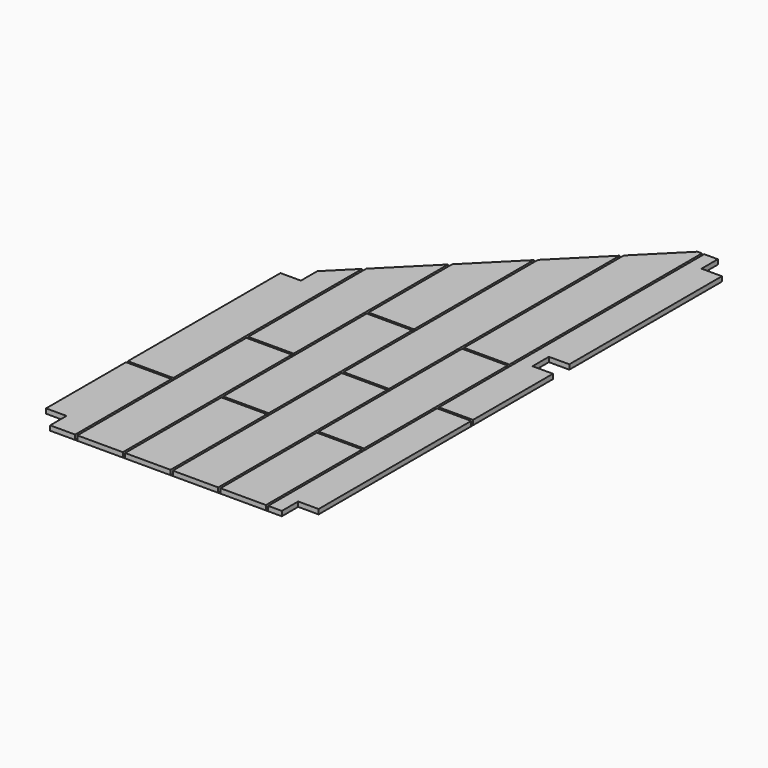
from build123d import *

# Parameters (mm, degrees)
F0_W     = 20
F0_H     = 93
F0_H_2   = 79
F0_H_3   = 53
F0_H_4   = 1
F0_W_2   = 15
F0_W_3   = 2
F0_H_5   = 9
F0_W_4   = 1
F0_W_5   = 6
F1_DEPTH = 0.1
F2_DEPTH = 2


# Not quite as in the source:
# - a feature names something its author has since deleted; it is built from what else it names


with BuildPart() as f1:
    # F0 (on Top) → F1 (new body)
    with BuildSketch(Plane.XY):
        Polygon((-134.4656153619, 144.6975417137), (-143.4656153619, 144.6975417137), (-143.4656153619, 104.6975417137), (-143.4656153619, 95.6975417137), (-143.4656153619, 64.6975417137), (-143.4656153619, 60.6975417137), (-123.4656153619, 60.6975417137), (-123.4656153619, 164.6975417137), (-134.4656153619, 153.6975417137), align=None)
        Polygon((-123.4656153619, 6.6975417137), (-123.4656153619, 59.6975417137), (-143.4656153619, 59.6975417137), (-143.4656153619, 55.6975417137), (-143.4656153619, 15.6975417137), (-134.4656153619, 15.6975417137), (-134.4656153619, 6.6975417137), align=None)
        with Locations((-112.4656153619, 53.1975417137)):
            Rectangle(F0_W, F0_H)
        Polygon((-102.4656153619, 185.6975417137), (-122.4656153619, 165.6975417137), (-122.4656153619, 100.6975417137), (-102.4656153619, 100.6975417137), align=None)
        Polygon((-81.4656153619, 140.6975417137), (-81.4656153619, 206.6975417137), (-101.4656153619, 186.6975417137), (-101.4656153619, 140.6975417137), align=None)
        with Locations((-91.4656153619, 100.1975417137)):
            Rectangle(F0_W, F0_H_2)
        with Locations((-91.4656153619, 33.1975417137)):
            Rectangle(F0_W, F0_H_3)
        Polygon((-60.4656153619, 100.6975417137), (-60.4656153619, 227.6975417137), (-80.4656153619, 207.6975417137), (-80.4656153619, 100.6975417137), align=None)
        with Locations((-70.4656153619, 53.1975417137)):
            Rectangle(F0_W, F0_H)
        Polygon((-41.4656153619, 237.6975417137), (-41.4656153619, 246.6975417137), (-59.4656153619, 228.6975417137), (-59.4656153619, 140.6975417137), (-39.4656153619, 140.6975417137), (-39.4656153619, 237.6975417137), align=None)
        with Locations((-49.4656153619, 100.1975417137)):
            Rectangle(F0_W, F0_H_2)
        with Locations((-49.4656153619, 33.1975417137)):
            Rectangle(F0_W, F0_H_3)
        with Locations((-133.4656153619, 60.1975417137)):
            Rectangle(F0_W, F0_H_4)
        Polygon((-122.4656153619, 165.6975417137), (-123.4656153619, 164.6975417137), (-123.4656153619, 60.6975417137), (-123.4656153619, 59.6975417137), (-123.4656153619, 6.6975417137), (-122.4656153619, 6.6975417137), (-122.4656153619, 99.6975417137), (-122.4656153619, 100.6975417137), align=None)
        with Locations((-112.4656153619, 100.1975417137)):
            Rectangle(F0_W, F0_H_4)
        Polygon((-101.4656153619, 186.6975417137), (-102.4656153619, 185.6975417137), (-102.4656153619, 100.6975417137), (-102.4656153619, 99.6975417137), (-102.4656153619, 6.6975417137), (-101.4656153619, 6.6975417137), (-101.4656153619, 59.6975417137), (-101.4656153619, 60.6975417137), (-101.4656153619, 139.6975417137), (-101.4656153619, 140.6975417137), align=None)
        with Locations((-91.4656153619, 140.1975417137)):
            Rectangle(F0_W, F0_H_4)
        Polygon((-80.4656153619, 100.6975417137), (-80.4656153619, 207.6975417137), (-81.4656153619, 206.6975417137), (-81.4656153619, 140.6975417137), (-81.4656153619, 139.6975417137), (-81.4656153619, 60.6975417137), (-81.4656153619, 59.6975417137), (-81.4656153619, 6.6975417137), (-80.4656153619, 6.6975417137), (-80.4656153619, 99.6975417137), align=None)
        with Locations((-70.4656153619, 100.1975417137)):
            Rectangle(F0_W, F0_H_4)
        Polygon((-59.4656153619, 140.6975417137), (-59.4656153619, 228.6975417137), (-60.4656153619, 227.6975417137), (-60.4656153619, 100.6975417137), (-60.4656153619, 99.6975417137), (-60.4656153619, 6.6975417137), (-59.4656153619, 6.6975417137), (-59.4656153619, 59.6975417137), (-59.4656153619, 60.6975417137), (-59.4656153619, 139.6975417137), align=None)
        with Locations((-49.4656153619, 60.1975417137)):
            Rectangle(F0_W, F0_H_4)
        with Locations((-49.4656153619, 140.1975417137)):
            Rectangle(F0_W, F0_H_4)
        with Locations((-91.4656153619, 60.1975417137)):
            Rectangle(F0_W, F0_H_4)
        Polygon((-38.4656153619, 237.6975417137), (-39.4656153619, 237.6975417137), (-39.4656153619, 140.6975417137), (-39.4656153619, 139.6975417137), (-39.4656153619, 60.6975417137), (-39.4656153619, 59.6975417137), (-39.4656153619, 6.6975417137), (-38.4656153619, 6.6975417137), (-38.4656153619, 99.6975417137), (-38.4656153619, 100.6975417137), align=None)
        Polygon((-23.4656153619, 99.6975417137), (-38.4656153619, 99.6975417137), (-38.4656153619, 6.6975417137), (-32.4656153619, 6.6975417137), (-32.4656153619, 15.6975417137), (-23.4656153619, 15.6975417137), align=None)
        Polygon((-32.4656153619, 237.6975417137), (-38.4656153619, 237.6975417137), (-38.4656153619, 100.6975417137), (-23.4656153619, 100.6975417137), (-23.4656153619, 144.6975417137), (-32.4656153619, 144.6975417137), (-32.4656153619, 153.6975417137), (-23.4656153619, 153.6975417137), (-23.4656153619, 237.6975417137), align=None)
        with Locations((-30.9656153619, 100.1975417137)):
            Rectangle(F0_W_2, F0_H_4)
        with Locations((-40.4656153619, 242.1975417137)):
            Rectangle(F0_W_3, F0_H_5)
        with Locations((-38.9656153619, 242.1975417137)):
            Rectangle(F0_W_4, F0_H_5)
        with Locations((-35.4656153619, 242.1975417137)):
            Rectangle(F0_W_5, F0_H_5)
    extrude(amount=-F1_DEPTH)

    # F0 (on Top) → F2 (join)
    with BuildSketch(Plane.XY):
        Polygon((-134.4656153619, 144.6975417137), (-143.4656153619, 144.6975417137), (-143.4656153619, 104.6975417137), (-143.4656153619, 95.6975417137), (-143.4656153619, 64.6975417137), (-143.4656153619, 60.6975417137), (-123.4656153619, 60.6975417137), (-123.4656153619, 164.6975417137), (-134.4656153619, 153.6975417137), align=None)
        Polygon((-123.4656153619, 6.6975417137), (-123.4656153619, 59.6975417137), (-143.4656153619, 59.6975417137), (-143.4656153619, 55.6975417137), (-143.4656153619, 15.6975417137), (-134.4656153619, 15.6975417137), (-134.4656153619, 6.6975417137), align=None)
        with Locations((-112.4656153619, 53.1975417137)):
            Rectangle(F0_W, F0_H)
        Polygon((-102.4656153619, 185.6975417137), (-122.4656153619, 165.6975417137), (-122.4656153619, 100.6975417137), (-102.4656153619, 100.6975417137), align=None)
        Polygon((-81.4656153619, 140.6975417137), (-81.4656153619, 206.6975417137), (-101.4656153619, 186.6975417137), (-101.4656153619, 140.6975417137), align=None)
        with Locations((-91.4656153619, 100.1975417137)):
            Rectangle(F0_W, F0_H_2)
        with Locations((-91.4656153619, 33.1975417137)):
            Rectangle(F0_W, F0_H_3)
        with Locations((-70.4656153619, 53.1975417137)):
            Rectangle(F0_W, F0_H)
        Polygon((-60.4656153619, 100.6975417137), (-60.4656153619, 227.6975417137), (-80.4656153619, 207.6975417137), (-80.4656153619, 100.6975417137), align=None)
        Polygon((-41.4656153619, 237.6975417137), (-41.4656153619, 246.6975417137), (-59.4656153619, 228.6975417137), (-59.4656153619, 140.6975417137), (-39.4656153619, 140.6975417137), (-39.4656153619, 237.6975417137), align=None)
        with Locations((-49.4656153619, 100.1975417137)):
            Rectangle(F0_W, F0_H_2)
        with Locations((-49.4656153619, 33.1975417137)):
            Rectangle(F0_W, F0_H_3)
        Polygon((-23.4656153619, 99.6975417137), (-38.4656153619, 99.6975417137), (-38.4656153619, 6.6975417137), (-32.4656153619, 6.6975417137), (-32.4656153619, 15.6975417137), (-23.4656153619, 15.6975417137), align=None)
        Polygon((-32.4656153619, 237.6975417137), (-38.4656153619, 237.6975417137), (-38.4656153619, 100.6975417137), (-23.4656153619, 100.6975417137), (-23.4656153619, 144.6975417137), (-32.4656153619, 144.6975417137), (-32.4656153619, 153.6975417137), (-23.4656153619, 153.6975417137), (-23.4656153619, 237.6975417137), align=None)
        with Locations((-40.4656153619, 242.1975417137)):
            Rectangle(F0_W_3, F0_H_5)
        with Locations((-35.4656153619, 242.1975417137)):
            Rectangle(F0_W_5, F0_H_5)
    extrude(amount=F2_DEPTH)


solid = f1.part
